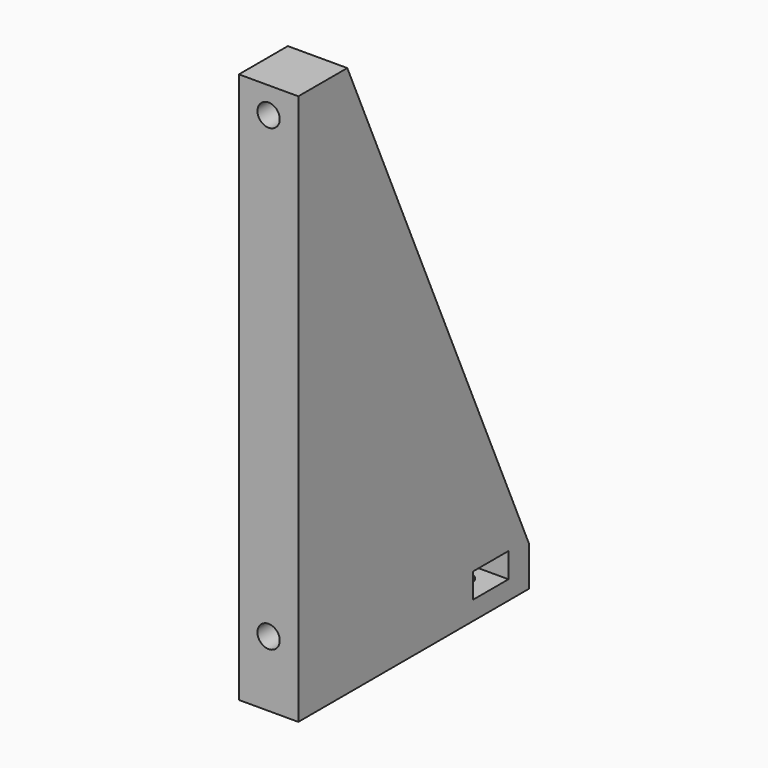
from build123d import *

# Parameters (mm, degrees)
F1_DEPTH  = 13.6
F3_D      = 5.1
F5_DEPTH  = 12
F6_DEPTH  = 25
F7_DEPTH  = 15
F8_D      = 5.1
F9_W      = 5.1
F9_H      = 5.7
F10_DEPTH = 25
F4_W      = 6.8
F4_H      = 4
F11_DEPTH = 25
F12_DEPTH = 25


# Not quite as in the source:
# - a feature names something its author has since deleted; it is built from what else it names


with BuildPart() as f1:
    # F0 (on Right) → F1 (new body)
    with BuildSketch(Plane.YZ):
        Polygon((-70, 0), (0, 0), (-56, 126), (-70, 126), align=None)
        Polygon((-70, 126), (-56, 126), (-60, 135), (-70, 135), align=None)
    extrude(amount=F1_DEPTH)

    # F3 (through all)
    with Locations(Plane.XZ.offset(70)):
        with Locations((6.8, 15), (6.8, 120)):
            Hole(F3_D / 2)

    # F4 (on face) → F5 (cut)
    with BuildSketch(Plane(origin=(0, 0, 0), x_dir=(1, 0, 0), z_dir=(0, 0, -1))):
        with BuildLine():
            ThreePointArc((9.35, 55), (8.603122292, 56.803122292), (6.8, 57.55))
            Line((6.8, 57.55), (6.8, 55))
            Line((6.8, 55), (6.8, 52.45))
            ThreePointArc((6.8, 52.45), (8.603122292, 53.196877708), (9.35, 55))
        make_face()
        with BuildLine():
            ThreePointArc((9.35, 15), (8.603122292, 16.803122292), (6.8, 17.55))
            ThreePointArc((6.8, 17.55), (4.996877708, 13.196877708), (9.35, 15))
        make_face()
        with BuildLine():
            Line((6.8, 55), (6.8, 57.55))
            ThreePointArc((6.8, 57.55), (4.25, 55), (6.8, 52.45))
            Line((6.8, 52.45), (6.8, 55))
        make_face()
    extrude(amount=-F5_DEPTH, mode=Mode.SUBTRACT)

    # F2 (on face) → F6 (join)
    with BuildSketch(Plane.XZ.offset(70)):
        Polygon((11.9, 122.9444863729), (6.8, 125.8889727457), (1.7, 122.9444863729), (1.7, 117.0555136271), (6.8, 114.1110272543), (11.9, 117.0555136271), align=None)
    extrude(amount=-F6_DEPTH)

    # F7 (cut): a face of the model
    f7_faces = [f1.faces().sort_by_distance(p)[0] for p in [
        (6.8, -45, 120),
    ]]
    extrude(f7_faces, amount=-F7_DEPTH, mode=Mode.SUBTRACT)

    # F8 (through all)
    with Locations(Plane.XZ.offset(70)):
        with Locations((6.8, 120)):
            Hole(F8_D / 2)

    # F9 (on face) → F10 (cut)
    with BuildSketch(Plane(origin=(0, 0, 0), x_dir=(0, -1, 0), z_dir=(-1, 0, 0))):
        with Locations((12.45, 7.15)):
            Rectangle(F9_W, F9_H)
        with Locations((17.55, 7.15)):
            Rectangle(F9_W, F9_H)
    extrude(amount=-F10_DEPTH, mode=Mode.SUBTRACT)

    # F4 (on face) → F11 (cut)
    with BuildSketch(Plane(origin=(0, 0, 0), x_dir=(1, 0, 0), z_dir=(0, 0, -1))):
        with Locations((10.2, 2)):
            Rectangle(F4_W, F4_H)
        with Locations((3.4, 2)):
            Rectangle(F4_W, F4_H)
    extrude(amount=-F11_DEPTH, mode=Mode.SUBTRACT)

    # F0 (on Right) → F12 (cut)
    with BuildSketch(Plane.YZ):
        Polygon((-70, 126), (-56, 126), (-60, 135), (-70, 135), align=None)
    extrude(amount=F12_DEPTH, mode=Mode.SUBTRACT)


solid = f1.part
